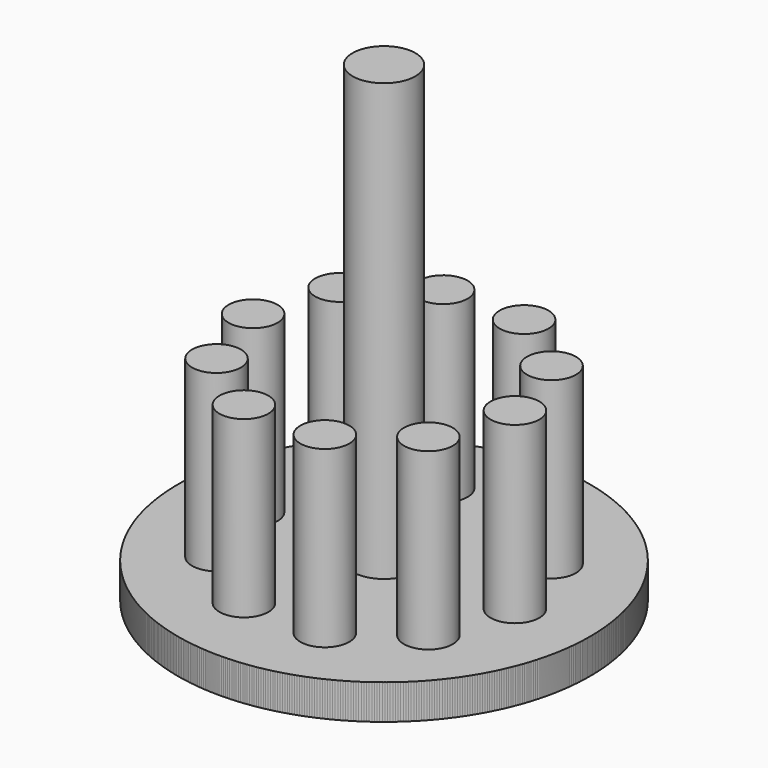
from build123d import *

# Parameters (mm, degrees)
F0_R     = 29.972
F1_DEPTH = 5.08
F2_R     = 3.556
F3_DEPTH = 25.4
F4_COUNT = 10
F5_R     = 4.572
F6_DEPTH = 63.5


# Not quite as in the source:
# - the program builds the solid bodies; features that only make, move or delete a surface that nothing else refers to are left out


with BuildPart() as f1:
    # F0 (on Top) → F1 (new body)
    with BuildSketch(Plane.XY):
        Circle(F0_R)
    extrude(amount=F1_DEPTH)

    # F2 (on face) → F3 (join)
    with BuildSketch(Plane.XY.offset(5.08)):
        with Locations((-19.05, 0)):
            Circle(F2_R)
    extrude(amount=F3_DEPTH)


with BuildPart() as f4_1:
    # F4: instance of F1
    add(f1.part.rotate(Axis((0, 0, 5.08), (0, 0, -1)), 1 * 360 / F4_COUNT))


with BuildPart() as f4_2:
    # F4: instance of F1
    add(f1.part.rotate(Axis((0, 0, 5.08), (0, 0, -1)), 2 * 360 / F4_COUNT))


with BuildPart() as f4_3:
    # F4: instance of F1
    add(f1.part.rotate(Axis((0, 0, 5.08), (0, 0, -1)), 3 * 360 / F4_COUNT))


with BuildPart() as f4_4:
    # F4: instance of F1
    add(f1.part.rotate(Axis((0, 0, 5.08), (0, 0, -1)), 4 * 360 / F4_COUNT))


with BuildPart() as f4_5:
    # F4: instance of F1
    add(f1.part.rotate(Axis((0, 0, 5.08), (0, 0, -1)), 5 * 360 / F4_COUNT))


with BuildPart() as f4_6:
    # F4: instance of F1
    add(f1.part.rotate(Axis((0, 0, 5.08), (0, 0, -1)), 6 * 360 / F4_COUNT))


with BuildPart() as f4_7:
    # F4: instance of F1
    add(f1.part.rotate(Axis((0, 0, 5.08), (0, 0, -1)), 7 * 360 / F4_COUNT))


with BuildPart() as f4_8:
    # F4: instance of F1
    add(f1.part.rotate(Axis((0, 0, 5.08), (0, 0, -1)), 8 * 360 / F4_COUNT))


with BuildPart() as f4_9:
    # F4: instance of F1
    add(f1.part.rotate(Axis((0, 0, 5.08), (0, 0, -1)), 9 * 360 / F4_COUNT))


with BuildPart() as f1_1:
    add(f1.part)

    # F5 (on face) → F6 (join)
    with BuildSketch(Plane.XY.offset(5.08)):
        Circle(F5_R)
    extrude(amount=F6_DEPTH)


solid = Compound([f4_1.part, f4_2.part, f4_3.part, f4_4.part, f4_5.part, f4_6.part, f4_7.part, f4_8.part, f4_9.part, f1_1.part])
